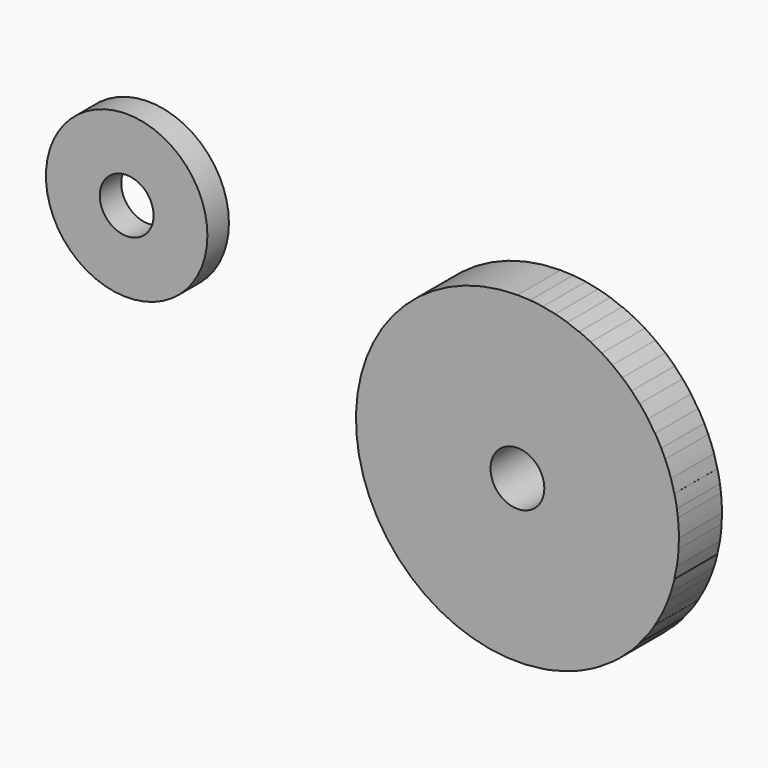
from build123d import *

# Parameters (mm, degrees)
F0_R     = 6.35
F1_DEPTH = 12.7
F2_R     = 19.05
F2_R_2   = 6.35
F3_DEPTH = 6.35


# Not quite as in the source:
# - ends of sketch curves that miss each other by under 0.0002 mm in the source are joined
# - a feature names something its author has since deleted; it is built from what else it names


with BuildPart() as f1:
    # F0 (on Front) → F1 (new body)
    with BuildSketch(Plane.XZ):
        with BuildLine():
            Line((28.8364005243, 24.9012450452), (26.9407683632, 26.9407683632))
            ThreePointArc((26.9407683632, 26.9407683632), (25.8623084048, 27.9776876095), (24.7439706414, 28.9714672894))
            ThreePointArc((24.7439706414, 28.9714672894), (24.7438711101, 28.9715522968), (24.7437715786, 28.9716373038))
            Line((24.7437715786, 28.9716373038), (22.3946181123, 30.8235474857))
            ThreePointArc((22.3946181123, 30.8235474857), (21.167225878, 31.6789922287), (19.9071953157, 32.4855902619))
            Line((19.9071953157, 32.4855902619), (17.2970380401, 33.9473485716))
            ThreePointArc((17.2970380401, 33.9473485716), (15.9476707836, 34.6017600214), (14.5735950651, 35.2025613682))
            Line((14.5735950651, 35.2025613682), (14.5628412955, 35.1538197769))
            Line((14.5628412955, 35.1538197769), (11.7735474857, 36.2352532708))
            ThreePointArc((11.7735474857, 36.2352532708), (10.3418811399, 36.6695445089), (8.8942683629, 37.0472939672))
            Line((8.8942683629, 37.0472939672), (5.9973227219, 37.6250198694))
            ThreePointArc((5.9973227219, 37.6250198694), (4.4968617978, 37.8336917835), (2.9892915472, 37.9825504152))
            Line((2.9892915472, 37.9825504152), (0, 38.1))
            ThreePointArc((0, 38.1), (-37.9825504152, -2.9892915472), (5.960153118, -37.6309257767))
            ThreePointArc((5.960153118, -37.6309257767), (7.4344130557, -37.3676263966), (8.8971866639, -37.0465932235))
            Line((8.8971866639, -37.0465932235), (8.8889522061, -37.0282024699))
            Line((8.8889522061, -37.0282024699), (11.7735474857, -36.2352532708))
            ThreePointArc((11.7735474857, -36.2352532708), (13.5733548782, -35.6001971533), (15.3391019224, -34.8758075493))
            Line((15.3391019224, -34.8758075493), (17.2970380401, -33.9473485716))
            ThreePointArc((17.2970380401, -33.9473485716), (18.6188813116, -33.2407469637), (19.9119094402, -32.4827009721))
            Line((19.9119094402, -32.4827009721), (19.8866817155, -32.4544715762))
            Line((19.8866817155, -32.4544715762), (22.3946181123, -30.8235474857))
            ThreePointArc((22.3946181123, -30.8235474857), (23.5898681595, -29.91869182), (24.7485963101, -28.9675159563))
            Line((24.7485963101, -28.9675159563), (24.716211253, -28.9410193531))
            Line((24.716211253, -28.9410193531), (26.9407683632, -26.9407683632))
            ThreePointArc((26.9407683632, -26.9407683632), (27.9811639514, -25.8585472122), (28.9781187619, -24.7361806474))
            Line((28.9781187619, -24.7361806474), (28.9154423412, -24.6986999505))
            Line((28.9154423412, -24.6986999505), (30.8235474857, -22.3946181123))
            ThreePointArc((30.8235474857, -22.3946181123), (31.6798259077, -21.1659781361), (32.4871583117, -19.9046362646))
            Line((32.4871583117, -19.9046362646), (32.4683314442, -19.897454679))
            Line((32.4683314442, -19.897454679), (33.9473485716, -17.2970380401))
            ThreePointArc((33.9473485716, -17.2970380401), (34.7709520965, -15.5753295408), (35.5073030041, -13.8145370308))
            Line((35.5073030041, -13.8145370308), (36.2352532708, -11.7735474857))
            ThreePointArc((36.2352532708, -11.7735474857), (36.670535285, -10.3383674684), (37.0489977594, -8.8871685607))
            Line((37.0489977594, -8.8871685607), (36.998361761, -8.8841095345))
            Line((36.998361761, -8.8841095345), (37.6309257767, -5.960153118))
            ThreePointArc((37.6309257767, -5.960153118), (37.8769274813, -4.1168391485), (38.0326909965, -2.2637171999))
            Line((38.0326909965, -2.2637171999), (38.1, 0))
            ThreePointArc((38.1, 0), (38.0435762549, 2.0727531781), (37.8744721398, 4.1393671175))
            Line((37.8744721398, 4.1393671175), (37.6309257767, 5.960153118))
            ThreePointArc((37.6309257767, 5.960153118), (37.3676263966, 7.4344130557), (37.0465932235, 8.8971866639))
            Line((37.0465932235, 8.8971866639), (37.0282024699, 8.8889522061))
            Line((37.0282024699, 8.8889522061), (36.2352532708, 11.7735474857))
            ThreePointArc((36.2352532708, 11.7735474857), (35.6001971533, 13.5733548782), (34.8758075493, 15.3391019224))
            Line((34.8758075493, 15.3391019224), (33.9473485716, 17.2970380401))
            ThreePointArc((33.9473485716, 17.2970380401), (33.24052825, 18.6192717812), (32.4822331625, 19.9126725674))
            Line((32.4822331625, 19.9126725674), (32.4491315845, 19.8832171692))
            Line((32.4491315845, 19.8832171692), (30.8235474857, 22.3946181123))
            ThreePointArc((30.8235474857, 22.3946181123), (29.8562915276, 23.6687949887), (28.8364005243, 24.9012450452))
        make_face()
        Circle(F0_R, mode=Mode.SUBTRACT)
    extrude(amount=F1_DEPTH)


with BuildPart() as f3:
    # F2 (on Front) → F3 (new body)
    with BuildSketch(Plane.XZ):
        with Locations((-97.2904128466, 22.4488124817)):
            Circle(F2_R)
        with Locations((-97.2904128466, 22.4488124817)):
            Circle(F2_R_2, mode=Mode.SUBTRACT)
    extrude(amount=F3_DEPTH)


solid = Compound([f1.part, f3.part])
